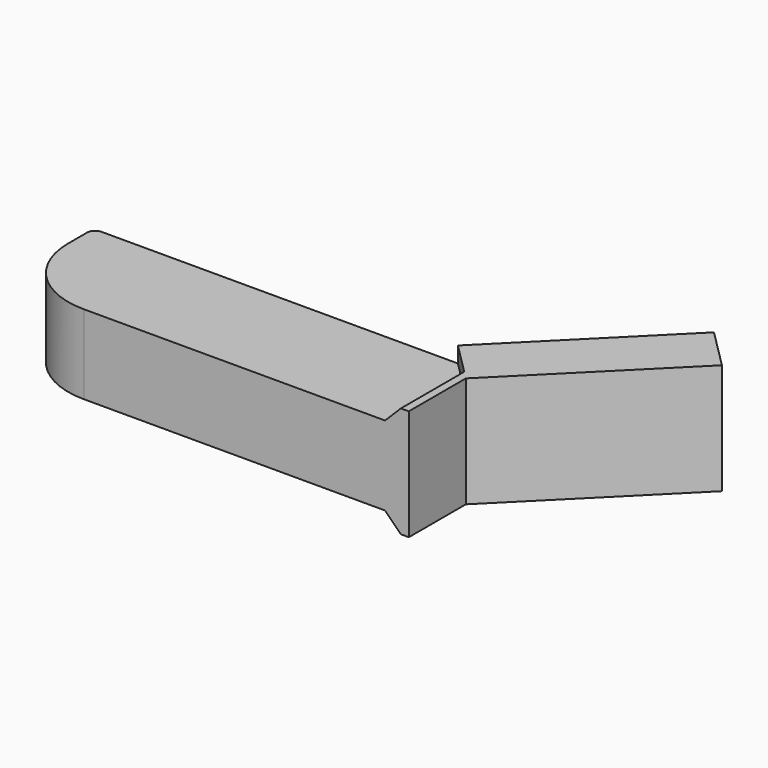
from build123d import *

# Parameters (mm, degrees)
F0_W          = 49.99736
F0_H          = 13.9954
F1_DEPTH      = 5
F1_DEPTH_BACK = 5
F2_R          = 1
F3_R          = 10
F4_W          = 13.9954
F4_H          = 13.9954
F5_DEPTH      = 1
F5_DEPTH_BACK = 5
F6_T4_DEPTH   = 39.7122298797
F6_T9_DEPTH   = 39.7122298797
F7_SIZE       = 5
F8_W          = 7.0710678119
F8_H          = 13.9954
F9_DEPTH      = 25.4


# Not quite as in the source:
# - a fillet or chamfer that OpenCascade refuses, or shapes differently, is made with other operations: its cross-section is extruded or revolved along the edge and cut away or added


with BuildPart() as f1:
    # F0 (on Top) → F1 (new body, two sides)
    with BuildSketch(Plane.XY) as f1_sk:
        Rectangle(F0_W, F0_H)
    extrude(amount=F1_DEPTH)
    extrude(f1_sk.sketch, amount=-F1_DEPTH_BACK)

    # F2
    f2_edges = [f1.edges().sort_by_distance(p)[0] for p in [
        (-24.99868, 6.9977, 0),
    ]]
    fillet(f2_edges, radius=F2_R)

    # F3
    f3_edges = [f1.edges().sort_by_distance(p)[0] for p in [
        (-24.99868, -6.9977, 0),
    ]]
    fillet(f3_edges, radius=F3_R)

    # F4 (on face) → F5 (join, two sides)
    with BuildSketch(Plane.YZ.offset(24.99868)) as f5_sk:
        Rectangle(F4_W, F4_H)
    extrude(amount=F5_DEPTH)
    extrude(f5_sk.sketch, amount=-F5_DEPTH_BACK)

    # F6: chamfer of 5 on 2 edges, made by hand


with BuildPart() as f6_tool2:
    # F6_s3 → F6_t4 (new body)
    with BuildSketch(Plane.XZ.offset(-19.8561149398)):
        Polygon((19.99868, 1.9977), (24.99868, 6.9977), (19.99868, 6.9977), align=None)
    extrude(amount=F6_T4_DEPTH)

    split(bisect_by=Plane.XY.offset(5), keep=Keep.TOP)


with BuildPart() as f1_1:
    add(f1.part)

    # F6_t1: cut F6_tool2
    add(f6_tool2.part, mode=Mode.SUBTRACT)


with BuildPart() as f6_tool7:
    # F6_s8 → F6_t9 (new body)
    with BuildSketch(Plane.XZ.offset(19.8561149398)):
        Polygon((19.99868, -1.9977), (24.99868, -6.9977), (19.99868, -6.9977), align=None)
    extrude(amount=-F6_T9_DEPTH)

    split(bisect_by=Plane.XY.offset(-5), keep=Keep.BOTTOM)


with BuildPart() as f1_2:
    add(f1_1.part)

    # F6_t6: cut F6_tool7
    add(f6_tool7.part, mode=Mode.SUBTRACT)

    # F7
    f7_edges = [f1_2.edges().sort_by_distance(p)[0] for p in [
        (25.99868, 6.9977, 0),
    ]]
    chamfer(f7_edges, length=F7_SIZE)

    # F8 (on face) → F9 (join)
    with BuildSketch(Plane(origin=(13.99819, 13.99819, 0), x_dir=(-0.7071067812, 0.7071067812, 0), z_dir=(0.7071067812, 0.7071067812, 0))):
        with Locations((-13.4357218072, 0)):
            Rectangle(F8_W, F8_H)
    extrude(amount=F9_DEPTH)


solid = f1_2.part
